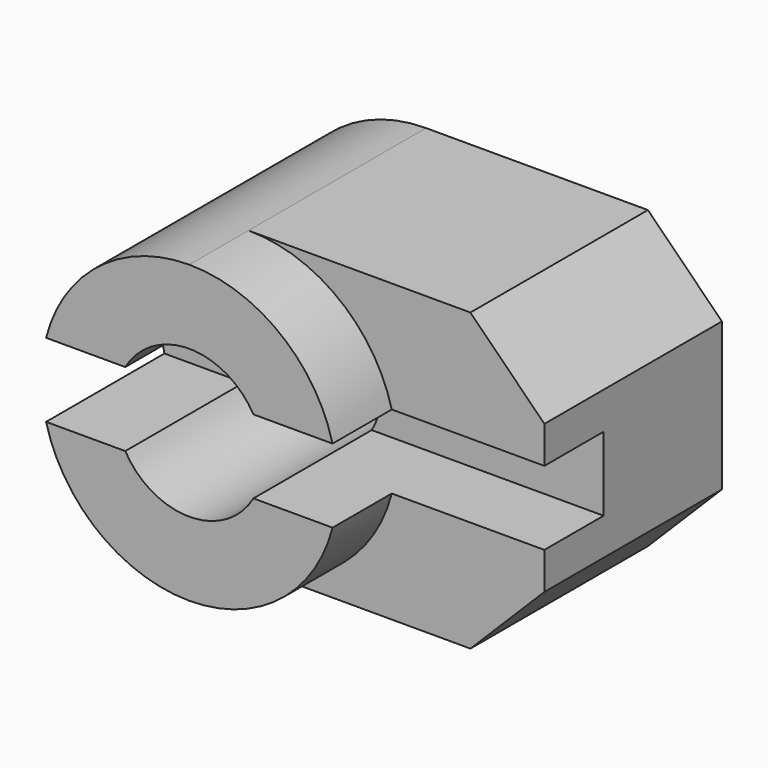
from build123d import *

# Parameters (mm, degrees)
F0_W          = 30
F0_H          = 20
F1_DEPTH      = 15
F2_R          = 5
F3_DEPTH      = 5
F4_DEPTH      = 15.001
F5_DEPTH      = 15.001
F7_DEPTH      = 5
F7_DEPTH_BACK = 10
F8_SIZE       = 5


with BuildPart() as f1:
    # F0 (on Front) → F1 (new body)
    with BuildSketch(Plane.XZ):
        with Locations((15, 10)):
            Rectangle(F0_W, F0_H)
    extrude(amount=F1_DEPTH)

    # F2 (on face) → F3 (join)
    with BuildSketch(Plane.XZ.offset(15)):
        with BuildLine():
            ThreePointArc((10, 0), (17.071068, 2.928932), (20, 10))
            ThreePointArc((20, 10), (17.071068, 17.071068), (10, 20))
            ThreePointArc((10, 20), (2.928932, 17.071068), (0, 10))
            ThreePointArc((0, 10), (2.928932, 2.928932), (10, 0))
        make_face()
        with Locations((10, 10)):
            Circle(F2_R, mode=Mode.SUBTRACT)
    extrude(amount=F3_DEPTH)

    # F4 (cut, through all): faces of the model
    f4_faces = [f1.faces().sort_by_distance(p)[0] for p in [
        (2.233679, -15, 17.766321),
        (2.233679, -15, 2.233679),
    ]]
    extrude(f4_faces, amount=-F4_DEPTH, mode=Mode.SUBTRACT)

    # F5 (cut, through all): a face of the model
    f5_faces = [f1.faces().sort_by_distance(p)[0] for p in [
        (10, -15, 10),
    ]]
    extrude(f5_faces, amount=-F5_DEPTH, mode=Mode.SUBTRACT)

    # F6 (on face) → F7 (cut, two sides)
    with BuildSketch(Plane.XZ.offset(15)) as f7_sk:
        with BuildLine():
            Line((30, 7.5), (30, 12.5))
            Line((30, 12.5), (19.682458, 12.5))
            ThreePointArc((19.682458, 12.5), (20, 10), (19.682458, 7.5))
            Line((19.682458, 7.5), (30, 7.5))
        make_face()
        with BuildLine():
            ThreePointArc((19.682458, 7.5), (20, 10), (19.682458, 12.5))
            Line((19.682458, 12.5), (0, 12.5))
            Line((0, 12.5), (0, 7.5))
            Line((0, 7.5), (19.682458, 7.5))
        make_face()
    extrude(amount=-F7_DEPTH, mode=Mode.SUBTRACT)
    extrude(f7_sk.sketch, amount=F7_DEPTH_BACK, mode=Mode.SUBTRACT)

    # F8
    f8_edges = [f1.edges().sort_by_distance(p)[0] for p in [
        (30, -7.5, 20),
        (30, -7.5, 0),
    ]]
    chamfer(f8_edges, length=F8_SIZE)


solid = f1.part
